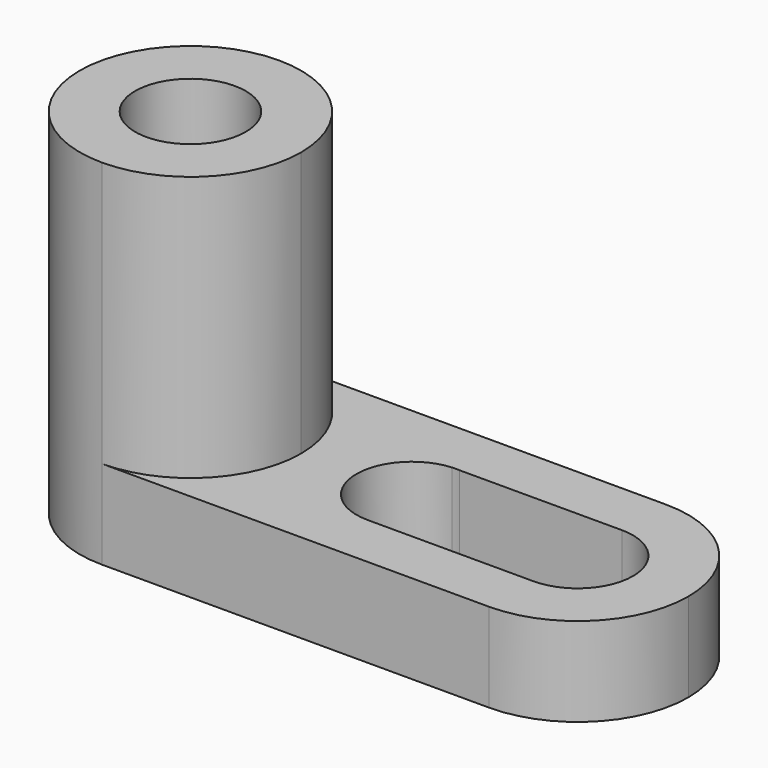
from build123d import *

# Parameters (mm, degrees)
F1_DEPTH = 25.4
F2_R     = 6.35
F3_DEPTH = 50.8
F4_R     = 12.69999
F6_DEPTH = 25.4


# Not quite as in the source:
# - a fillet or chamfer is up to 0.001 mm smaller than in the source, because OpenCascade refuses the exact size


with BuildPart() as f1:
    # F0 (on Front) → F1 (new body)
    with BuildSketch(Plane.XZ):
        Polygon((0, 40.6317008091), (0, 0), (69.85, 0), (69.85, 10.1959701541), (25.413833983, 10.1959701541), (25.413833983, 40.6317008091), align=None)
    extrude(amount=F1_DEPTH)

    # F2 (on face) → F3 (cut)
    with BuildSketch(Plane.XY.offset(40.6317008091)):
        with Locations((12.7069169915, -12.7)):
            Circle(F2_R)
    extrude(amount=-F3_DEPTH, mode=Mode.SUBTRACT)

    # F4 (radius 12.7 in the source; OpenCascade refuses exactly that, so slightly less here)
    f4_edges = [f1.edges().sort_by_distance(p)[0] for p in [
        (25.413834, -25.4, 25.413835),
        (25.413834, 0, 25.413835),
        (0, -25.4, 20.31585),
        (0, 0, 20.31585),
        (69.85, -25.4, 5.097985),
        (69.85, 0, 5.097985),
    ]]
    fillet(f4_edges, radius=F4_R)

    # F5 (on face) → F6 (cut)
    with BuildSketch(Plane.XY.offset(10.1959701541)):
        with BuildLine():
            Line((38.5519873755, -6.3651344446), (37.6653695389, -6.365856045))
            ThreePointArc((37.6653695389, -6.365856045), (31.7677992323, -12.9243723311), (38.113833983, -19.05))
            ThreePointArc((38.113833983, -19.05), (42.6039620435, -17.1901280605), (44.463833983, -12.7))
            ThreePointArc((44.463833983, -12.7), (42.7562888316, -8.3675511568), (38.5519873755, -6.3651344446))
        make_face()
        with BuildLine():
            ThreePointArc((38.5519873755, -6.3651344446), (38.1086658476, -6.3500021031), (37.6653695389, -6.365856045))
            Line((37.6653695389, -6.365856045), (38.5519873755, -6.3651344446))
        make_face()
        with BuildLine():
            ThreePointArc((44.463833983, -12.7), (42.6039620435, -17.1901280605), (38.113833983, -19.05))
            Line((38.113833983, -19.05), (57.15, -19.05))
            ThreePointArc((57.15, -19.05), (50.8000005258, -12.7025840679), (57.1448318647, -6.3500021031))
            Line((57.1448318647, -6.3500021031), (38.5519873755, -6.3651344446))
            ThreePointArc((38.5519873755, -6.3651344446), (42.7562888316, -8.3675511568), (44.463833983, -12.7))
        make_face()
        with BuildLine():
            ThreePointArc((57.1448318647, -6.3500021031), (50.8000005258, -12.7025840679), (57.15, -19.05))
            ThreePointArc((57.15, -19.05), (61.6401280605, -17.1901280605), (63.5, -12.7))
            ThreePointArc((63.5, -12.7), (61.6383004768, -8.2080450993), (57.1448318647, -6.3500021031))
        make_face()
    extrude(amount=-F6_DEPTH, mode=Mode.SUBTRACT)


solid = f1.part
